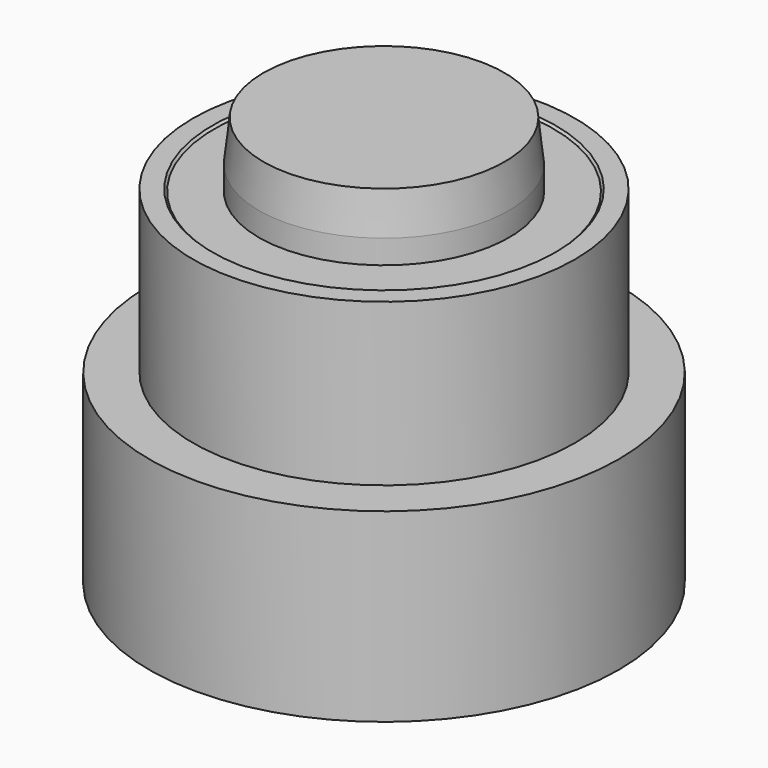
from build123d import *

# Parameters (mm, degrees)
F1_R     = 10
F2_DEPTH = 9.2
F3_R     = 37.5
F4_DEPTH = 29.6
F5_R     = 30.5
F6_DEPTH = 25.8
F7_R     = 26.905
F8_DEPTH = 0.35


# Not quite as in the source:
# - a fillet or chamfer that OpenCascade refuses, or shapes differently, is made with other operations: its cross-section is extruded or revolved along the edge and cut away or added


with BuildPart() as f2:
    # F1 (on Top) → F2 (new body)
    with BuildSketch(Plane.XY):
        Circle(F1_R)
    extrude(amount=F2_DEPTH)

    # F3 (on face) → F4 (join)
    with BuildSketch(Plane.XY.offset(9.2)):
        Circle(F3_R)
    extrude(amount=F4_DEPTH)

    # F5 (on face) → F6 (join)
    with BuildSketch(Plane.XY.offset(38.8)):
        Circle(F5_R)
    extrude(amount=F6_DEPTH)

    # F7 (on face) → F8 (cut)
    with BuildSketch(Plane.XY.offset(64.6)):
        Circle(F7_R)
    extrude(amount=-F8_DEPTH, mode=Mode.SUBTRACT)

    # F10: chamfer of 0.5 on 2 edges, made by hand


with BuildPart() as f10_tool2:
    # F10_s3 → F10_t4 (revolve)
    with BuildSketch(Plane.XZ):
        Polygon((27.405, 64.6), (26.905, 64.1), (26.905, 64.6), align=None)
    revolve(axis=Axis((0, 0, 64.6), (0, 0, 1)))

    split(bisect_by=Plane.XY.offset(64.25), keep=Keep.TOP)


with BuildPart() as f2_1:
    add(f2.part)

    # F10_t1: cut F10_tool2
    add(f10_tool2.part, mode=Mode.SUBTRACT)

    # F10_s6 → F10_t7 (revolve, cut)
    with BuildSketch(Plane.XZ):
        Polygon((10, 0.5), (9.5, 0), (10, 0), align=None)
    revolve(axis=Axis((0, 0, 0), (0, 0, 1)), mode=Mode.SUBTRACT)

    # F11 (on Front) → F12 (revolve)
    with BuildSketch(Plane.XZ):
        Polygon((0, 64.25), (0, 74.65), (-19.25, 74.65), (-19.975, 68.05), (-19.975, 64.25), align=None)
    revolve(axis=Axis((0, 0, 44.8884957004), (0, 0, -1)))


solid = f2_1.part
